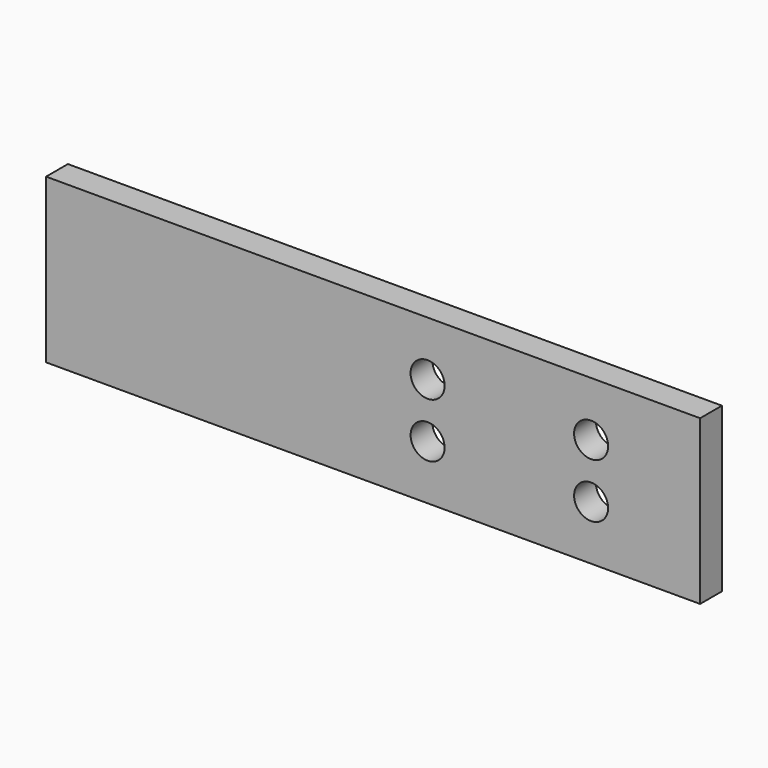
from build123d import *

# Parameters (mm, degrees)
F0_W     = 76.2
F0_H     = 19.05
F1_DEPTH = 1.5875
F2_R     = 1.984375
F2_R_2   = 1.9812
F3_DEPTH = 3.175
F4_DEPTH = 3.175


# Not quite as in the source:
# - a length typed as a fraction of an inch, garbled in the dataset ("3 / 203.2 mm" for 3/8 in), is restored


with BuildPart() as f1:
    # F0 (on Front) → F1 (new body, symmetric)
    with BuildSketch(Plane.XZ):
        Rectangle(F0_W, F0_H)
    extrude(amount=F1_DEPTH, both=True)

    # F2 (on face) → F3 (cut)
    with BuildSketch(Plane.XZ.offset(1.5875)):
        with Locations((6.35, 3.175)):
            Circle(F2_R)
        with Locations((6.35, -3.175)):
            Circle(F2_R_2)
        with Locations((25.4, 3.175)):
            Circle(F2_R)
        with Locations((25.4, -3.175)):
            Circle(F2_R_2)
    extrude(amount=-F3_DEPTH, mode=Mode.SUBTRACT)

    # F2 (on face) → F4 (cut)
    with BuildSketch(Plane.XZ.offset(1.5875)):
        with Locations((6.35, 3.175)):
            Circle(F2_R)
        with Locations((6.35, -3.175)):
            Circle(F2_R_2)
        with Locations((25.4, 3.175)):
            Circle(F2_R)
        with Locations((25.4, -3.175)):
            Circle(F2_R_2)
    extrude(amount=-F4_DEPTH, mode=Mode.SUBTRACT)


solid = f1.part
